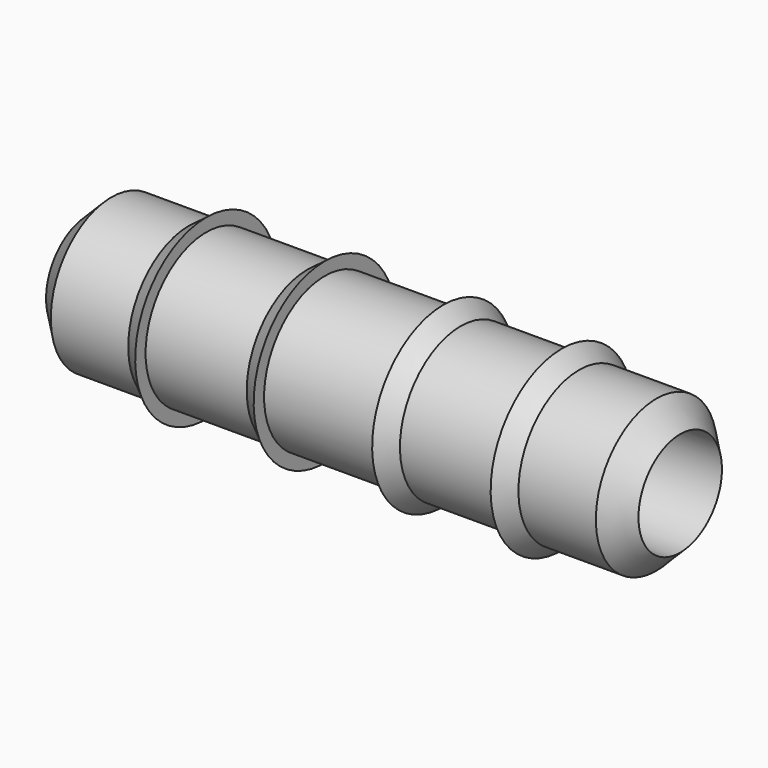
from build123d import *

# Parameters (mm, degrees)
F0_R     = 6.4
F1_DEPTH = 50
F4_R     = 4.4
F5_DEPTH = 50.001
F6_SIZE  = 1.99999


# Not quite as in the source:
# - a fillet or chamfer is up to 0.001 mm smaller than in the source, because OpenCascade refuses the exact size


with BuildPart() as f1:
    # F0 (on Right) → F1 (new body)
    with BuildSketch(Plane.YZ):
        Circle(F0_R)
    extrude(amount=F1_DEPTH)

    # F2 (on Front) → F3 (revolve)
    with BuildSketch(Plane.XZ):
        Polygon((10, 0), (10, 7.5), (0, 0), align=None)
        Polygon((20, 0), (20, 7.5), (10, 0), align=None)
        Polygon((40, 0), (30, 7.5), (30, 0), align=None)
        Polygon((50, 0), (40, 7.5), (40, 0), align=None)
    revolve(axis=Axis((25, 0, 0), (1, 0, 0)))

    # F4 (on face) → F5 (cut, through all)
    with BuildSketch(Plane(origin=(0, 0, 0), x_dir=(0, -1, 0), z_dir=(-1, 0, 0))):
        Circle(F4_R)
    extrude(amount=-F5_DEPTH, mode=Mode.SUBTRACT)

    # F6 (size 2 in the source; OpenCascade refuses exactly that, so slightly less here)
    f6_edges = [f1.edges().sort_by_distance(p)[0] for p in [
        (50, -6.4, 0),
        (0, -6.4, 0),
    ]]
    chamfer(f6_edges, length=F6_SIZE)


solid = f1.part
